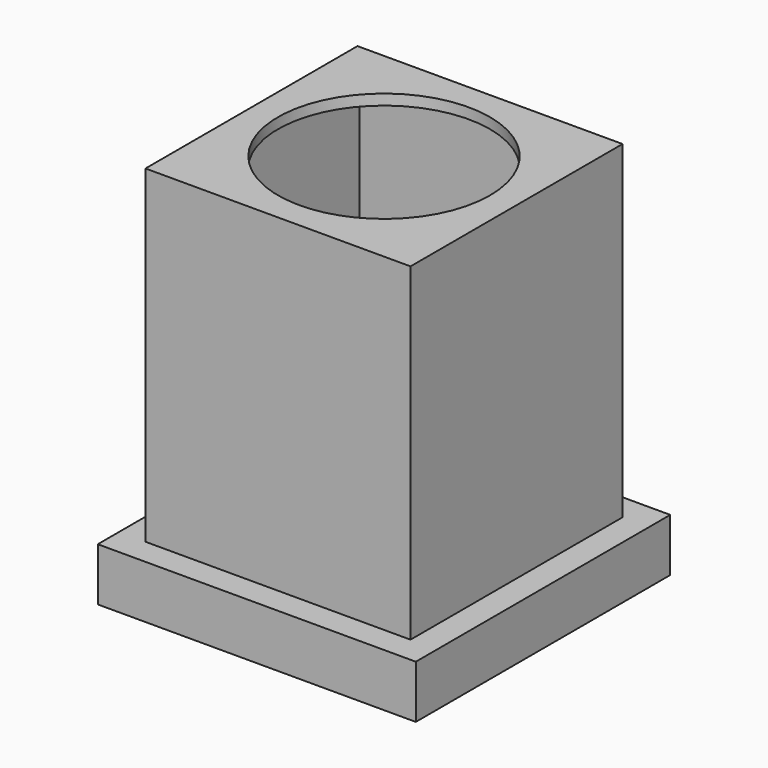
from build123d import *

# Parameters (mm, degrees)
F0_W      = 76.2
F0_H      = 76.2
F1_DEPTH  = 12.7
F2_W      = 63.5
F2_H      = 63.5
F3_DEPTH  = 76.2
F6_T      = -2.54
F7_W      = 63.5
F7_H      = 63.5
F8_DEPTH  = 2.54
F9_R      = 25.4
F10_DEPTH = 25.4


# Not quite as in the source:
# - a feature of the source that left no trace in its solid (it failed there, or was rolled back) is left out


with BuildPart() as f1:
    # F0 (on Top) → F1 (new body)
    with BuildSketch(Plane.XY):
        Rectangle(F0_W, F0_H)
    extrude(amount=F1_DEPTH)

    # F2 (on face) → F3 (join)
    with BuildSketch(Plane.XY.offset(12.7)):
        Rectangle(F2_W, F2_H)
    extrude(amount=F3_DEPTH)

    # F6
    f6_openings = [f1.faces().sort_by_distance(p)[0] for p in [
        (0, 0, 88.9),
    ]]
    offset(amount=F6_T, openings=f6_openings, kind=Kind.INTERSECTION)

    # F7 (on face) → F8 (join)
    with BuildSketch(Plane.XY.offset(88.9)):
        Rectangle(F7_W, F7_H)
    extrude(amount=F8_DEPTH)

    # F9 (on face) → F10 (cut)
    with BuildSketch(Plane.XY.offset(91.44)):
        Circle(F9_R)
    extrude(amount=-F10_DEPTH, mode=Mode.SUBTRACT)


solid = f1.part
